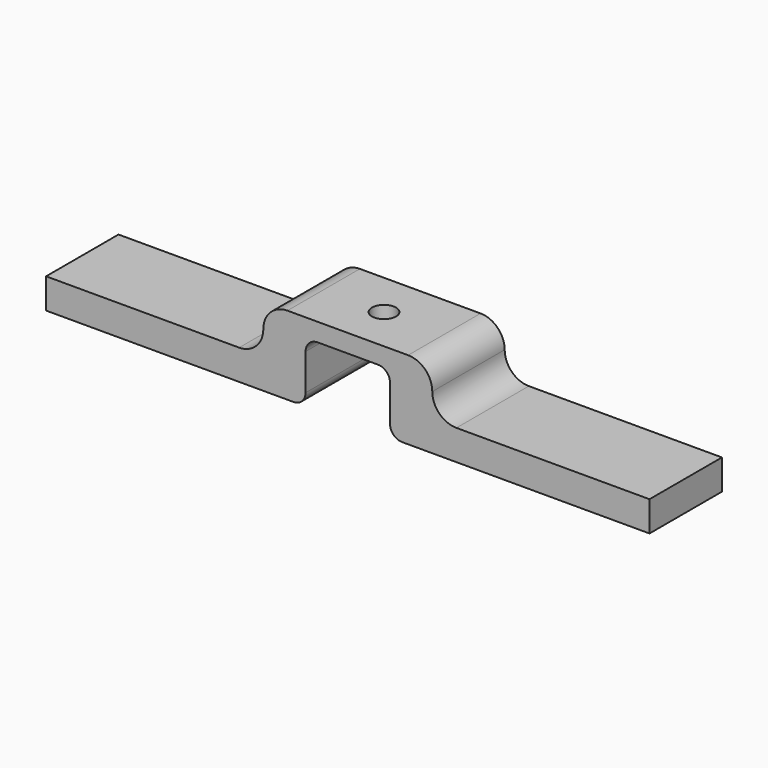
from build123d import *

# Parameters (mm, degrees)
F1_DEPTH = 19.05
F2_R     = 5.07999
F3_R     = 2.54
F4_DEPTH = 25.4
F5_R     = 2.54


# Not quite as in the source:
# - a fillet or chamfer is up to 0.001 mm smaller than in the source, because OpenCascade refuses the exact size


with BuildPart() as f1:
    # F0 (on Front) → F1 (new body)
    with BuildSketch(Plane.XZ):
        Polygon((17.78, -6.35), (17.78, 3.81), (-17.78, 3.81), (-17.78, -6.35), (-63.5, -6.35), (-63.5, -12.7), (-8.89, -12.7), (-8.89, 0), (8.89, 0), (8.89, -12.7), (63.5, -12.7), (63.5, -6.35), align=None)
    extrude(amount=F1_DEPTH)

    # F2 (radius 5.08 in the source; OpenCascade refuses exactly that, so slightly less here)
    f2_edges = [f1.edges().sort_by_distance(p)[0] for p in [
        (17.78, -9.525, 3.81),
        (17.78, -9.525, -6.35),
        (-17.78, -9.525, 3.81),
        (-17.78, -9.525, -6.35),
    ]]
    fillet(f2_edges, radius=F2_R)

    # F3 (on face) → F4 (cut)
    with BuildSketch(Plane.XY.offset(3.81)):
        with Locations((0, -9.525)):
            Circle(F3_R)
    extrude(amount=-F4_DEPTH, mode=Mode.SUBTRACT)

    # F5
    f5_edges = [f1.edges().sort_by_distance(p)[0] for p in [
        (8.89, -9.525, 0),
        (-8.89, -9.525, 0),
        (-8.89, -9.525, -12.7),
        (8.89, -9.525, -12.7),
    ]]
    fillet(f5_edges, radius=F5_R)


solid = f1.part
